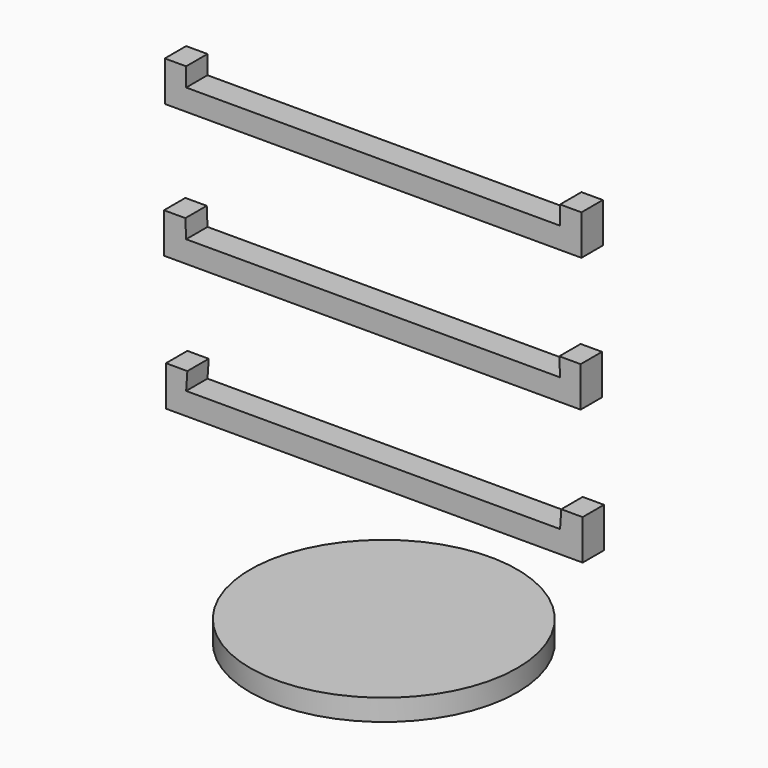
from build123d import *

# Parameters (mm, degrees)
F0_R     = 63.5
F1_DEPTH = 10.16
F5_DEPTH = 6.35


# Not quite as in the source:
# - the program builds the solid bodies; features that only make, move or delete a surface that nothing else refers to are left out


with BuildPart() as f1:
    # F0 (on Top) → F1 (new body)
    with BuildSketch(Plane.XY):
        Circle(F0_R)
    extrude(amount=F1_DEPTH)


with BuildPart() as f5:
    # F4 (on Front) → F5 (new body, symmetric)
    with BuildSketch(Plane.XZ):
        Polygon((-88.3273622656, 68.6497017741), (0, 68.6497017741), (0, 74.1204561174), (0, 79.2004561174), (-88.9, 79.2004561174), (-88.3273622656, 87.6997017741), (-98.4873622656, 87.6997017741), (-98.4873622656, 68.6497017741), align=None)
        Polygon((0, 74.1204561174), (0, 68.6497017741), (0.5726377344, 68.6497017741), (89.4726377344, 68.6497017741), (99.6326377344, 68.6497017741), (99.6326377344, 87.6997017741), (89.4726377344, 87.6997017741), (88.9, 79.2004561174), (0, 79.2004561174), align=None)
    extrude(amount=F5_DEPTH, both=True)


with BuildPart() as f5b:
    # F4 (on Front) → F5, piece 2 (new body, symmetric)
    with BuildSketch(Plane.XZ):
        Polygon((-88.9, 196.0404561174), (0, 196.0404561174), (88.9, 196.0404561174), (99.06, 196.0408687592), (99.06, 215.0904561174), (88.9, 215.0904561174), (88.9, 206.2004561174), (0, 206.2004561174), (-88.9, 206.2004561174), (-88.9, 215.0904561174), (-99.0599915385, 215.0904561174), (-99.0599915385, 196.0404561174), align=None)
    extrude(amount=F5_DEPTH, both=True)


with BuildPart() as f5c:
    # F4 (on Front) → F5, piece 3 (new body, symmetric)
    with BuildSketch(Plane.XZ):
        Polygon((-0.3752847338, 132.3706507683), (0, 132.3706507683), (0, 137.6204561174), (0, 142.7004561174), (-88.9, 142.7004561174), (-89.2752847338, 151.4206507683), (-99.4352847338, 151.4206507683), (-99.4352847338, 132.3706507683), (-89.2752847338, 132.3706507683), align=None)
        Polygon((0, 137.6204561174), (0, 132.3706507683), (88.5247152662, 132.3706507683), (98.6847152662, 132.3706507683), (98.6847152662, 151.4206507683), (88.5247152662, 151.4206507683), (88.9, 142.7004561174), (0, 142.7004561174), align=None)
    extrude(amount=F5_DEPTH, both=True)


solid = Compound([f1.part, f5.part, f5b.part, f5c.part])
